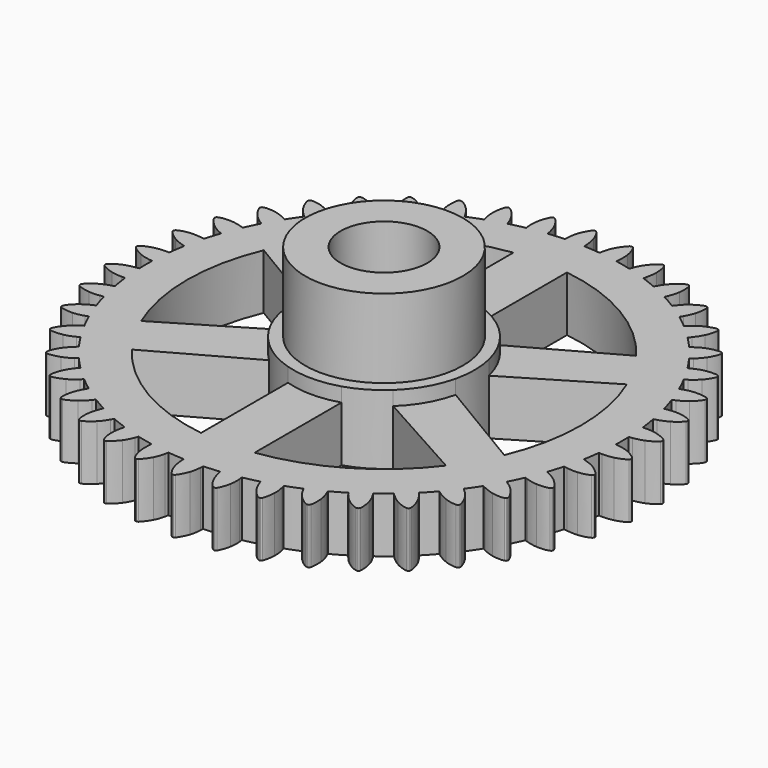
from build123d import *

# Parameters (mm, degrees)
F1_DEPTH  = 7
F2_R      = 4.1761413922
F3_DEPTH  = 25
F4_COUNT  = 42
F5_R      = 6.4823184413
F6_DEPTH  = 25
F7_R      = 30.25
F8_DEPTH  = 7
F10_DEPTH = 25
F11_R     = 5
F12_DEPTH = 1.8
F13_R     = 9.9
F13_R_2   = 5.0182312696
F14_DEPTH = 10
F15_R     = 10.7
F15_R_2   = 9.9
F16_DEPTH = 10
F17_R     = 12.382170164
F17_R_2   = 10
F18_DEPTH = 10
F17_R_3   = 5.5
F17_R_4   = 5.0182312696
F19_DEPTH = 91.7


with BuildPart() as f1:
    # F0 (on Top) → F1 (new body)
    with BuildSketch(Plane.XY):
        Polygon((0, 33.4545062297), (0, 33.4794496384), (-0.0728446466, 33.4794496384), align=None)
        with BuildLine():
            Line((0.0671612015, 33.4794496384), (0, 33.4794496384))
            Line((0, 33.4794496384), (0, 33.4545062297))
            Line((0, 33.4545062297), (0.2374699397, 33.3731919527))
            add(Edge.make_bspline(
                [(0.0671612015, 33.4794496384), (0.1192540142, 33.460955868), (0.1739978151, 33.4328680358), (0.2374699397, 33.3731919527)],
                knots=[0.0493061826, 0.0493061826, 0.0493061826, 0.0493061826, 0.1623395891, 0.1623395891, 0.1623395891, 0.1623395891], degree=3))
        make_face()
        Polygon((0.2374699397, 33.3731919527), (0, 33.4545062297), (0, 33.3731919527), align=None)
        with BuildLine():
            Line((0, 33.4545062297), (-0.0728446466, 33.4794496384))
            add(Edge.make_bspline(
                [(-0.0728446466, 33.4794496384), (-0.1154598232, 33.4657120562), (-0.1668077634, 33.4453793507), (-0.2365300603, 33.3731919527)],
                knots=[0.0695031824, 0.0695031824, 0.0695031824, 0.0695031824, 0.1811062055, 0.1811062055, 0.1811062055, 0.1811062055], degree=3))
            Line((-0.2365300603, 33.3731919527), (0, 33.3731919527))
            Line((0, 33.3731919527), (0, 33.4545062297))
        make_face()
        Polygon((0, 33.3731919527), (-0.2365300603, 33.3731919527), (0, 33.1028739042), align=None)
        with BuildLine():
            Line((0, 33.1028739042), (0.9666862315, 31.9980978966))
            add(Edge.make_bspline(
                [(0.2374699397, 33.3731919527), (0.4566645874, 33.1671065558), (0.7799529877, 32.5843005356), (0.9666862315, 31.9980978966)],
                knots=[0.1623395891, 0.1623395891, 0.1623395891, 0.1623395891, 0.5526891769, 0.5526891769, 0.5526891769, 0.5526891769], degree=3))
            Line((0.2374699397, 33.3731919527), (0, 33.3731919527))
            Line((0, 33.3731919527), (0, 33.1028739042))
        make_face()
        with BuildLine():
            add(Edge.make_bspline(
                [(-0.2365300603, 33.3731919527), (-0.4334827386, 33.1692758165), (-0.7770551927, 32.5515806531), (-0.9673137685, 31.9980978966)],
                knots=[0.1811062055, 0.1811062055, 0.1811062055, 0.1811062055, 0.4963642407, 0.4963642407, 0.4963642407, 0.4963642407], degree=3))
            Line((-0.9673137685, 31.9980978966), (0, 31.9980978966))
            Line((0, 31.9980978966), (0, 33.1028739042))
            Line((0, 33.1028739042), (-0.2365300603, 33.3731919527))
        make_face()
        Polygon((0, 31.9980978966), (0.9666862315, 31.9980978966), (0, 33.1028739042), align=None)
        with BuildLine():
            Line((0, 31.4007098089), (1.2083290596, 30.6544768805))
            add(Edge.make_bspline(
                [(0.9666862315, 31.9980978966), (1.1088668183, 31.5517572588), (1.1718801794, 31.1034474468), (1.2083290596, 30.6544768805)],
                knots=[0.5526891769, 0.5526891769, 0.5526891769, 0.5526891769, 0.8499053141, 0.8499053141, 0.8499053141, 0.8499053141], degree=3))
            Line((0.9666862315, 31.9980978966), (0, 31.9980978966))
            Line((0, 31.9980978966), (0, 31.4007098089))
        make_face()
        Polygon((0, 31.9980978966), (-0.9673137685, 31.9980978966), (0, 31.4007098089), align=None)
        with BuildLine():
            add(Edge.make_bspline(
                [(-0.9673137685, 31.9980978966), (-1.1457987858, 31.4788656937), (-1.1893575316, 31.0161446216), (-1.2146658644, 30.6501507258)],
                knots=[0.4963642407, 0.4963642407, 0.4963642407, 0.4963642407, 0.792113516, 0.792113516, 0.792113516, 0.792113516], degree=3))
            Line((-1.2146658644, 30.6501507258), (0, 30.6501507258))
            Line((0, 30.6501507258), (0, 31.4007098089))
            Line((0, 31.4007098089), (-0.9673137685, 31.9980978966))
        make_face()
        with BuildLine():
            Line((0, 30.6501507258), (1.2086794487, 30.6501507258))
            add(Edge.make_bspline(
                [(1.2083290596, 30.6544768805), (1.2084461294, 30.6530348357), (1.2085629252, 30.6515927842), (1.2086794487, 30.6501507258)],
                knots=[0.8499053141, 0.8499053141, 0.8499053141, 0.8499053141, 0.8508599401, 0.8508599401, 0.8508599401, 0.8508599401], degree=3))
            Line((1.2083290596, 30.6544768805), (0, 31.4007098089))
            Line((0, 31.4007098089), (0, 30.6501507258))
        make_face()
        with BuildLine():
            ThreePointArc((0, 30), (0.6251357368, 29.993486048), (1.25, 29.9739470207))
            add(Edge.make_bspline(
                [(1.2086794487, 30.6501507258), (1.2268837738, 30.4248597009), (1.2384418869, 30.1994033608), (1.25, 29.9739470207)],
                knots=[0.8508599401, 0.8508599401, 0.8508599401, 0.8508599401, 1, 1, 1, 1], degree=3))
            Line((1.2086794487, 30.6501507258), (0, 30.6501507258))
            Line((0, 30.6501507258), (0, 30))
        make_face()
        with BuildLine():
            add(Edge.make_bspline(
                [(-1.2146658644, 30.6501507258), (-1.2324554611, 30.3928882723), (-1.2412277305, 30.1834176465), (-1.25, 29.9739470207)],
                knots=[0.792113516, 0.792113516, 0.792113516, 0.792113516, 1, 1, 1, 1], degree=3))
            ThreePointArc((-1.25, 29.9739470207), (-0.6251357368, 29.993486048), (0, 30))
            Line((0, 30), (0, 30.6501507258))
            Line((0, 30.6501507258), (-1.2146658644, 30.6501507258))
        make_face()
    extrude(amount=F1_DEPTH)


with BuildPart() as f3:
    # F2 (on Top) → F3 (new body)
    with BuildSketch(Plane.XY):
        Circle(F2_R)
    extrude(amount=F3_DEPTH)

    # F5 (on face) → F6 (cut)
    with BuildSketch(Plane.XY.offset(25)):
        Circle(F5_R)
    extrude(amount=-F6_DEPTH, mode=Mode.SUBTRACT)


with BuildPart() as f4_1:
    # F4: instance of F1
    add(f1.part.rotate(Axis((0, 0, 25), (0, 0, 1)), 1 * 360 / F4_COUNT))


with BuildPart() as f4_2:
    # F4: instance of F1
    add(f1.part.rotate(Axis((0, 0, 25), (0, 0, 1)), 2 * 360 / F4_COUNT))


with BuildPart() as f4_3:
    # F4: instance of F1
    add(f1.part.rotate(Axis((0, 0, 25), (0, 0, 1)), 3 * 360 / F4_COUNT))


with BuildPart() as f4_4:
    # F4: instance of F1
    add(f1.part.rotate(Axis((0, 0, 25), (0, 0, 1)), 4 * 360 / F4_COUNT))


with BuildPart() as f4_5:
    # F4: instance of F1
    add(f1.part.rotate(Axis((0, 0, 25), (0, 0, 1)), 5 * 360 / F4_COUNT))


with BuildPart() as f4_6:
    # F4: instance of F1
    add(f1.part.rotate(Axis((0, 0, 25), (0, 0, 1)), 6 * 360 / F4_COUNT))


with BuildPart() as f4_7:
    # F4: instance of F1
    add(f1.part.rotate(Axis((0, 0, 25), (0, 0, 1)), 7 * 360 / F4_COUNT))


with BuildPart() as f4_8:
    # F4: instance of F1
    add(f1.part.rotate(Axis((0, 0, 25), (0, 0, 1)), 8 * 360 / F4_COUNT))


with BuildPart() as f4_9:
    # F4: instance of F1
    add(f1.part.rotate(Axis((0, 0, 25), (0, 0, 1)), 9 * 360 / F4_COUNT))


with BuildPart() as f4_10:
    # F4: instance of F1
    add(f1.part.rotate(Axis((0, 0, 25), (0, 0, 1)), 10 * 360 / F4_COUNT))


with BuildPart() as f4_11:
    # F4: instance of F1
    add(f1.part.rotate(Axis((0, 0, 25), (0, 0, 1)), 11 * 360 / F4_COUNT))


with BuildPart() as f4_12:
    # F4: instance of F1
    add(f1.part.rotate(Axis((0, 0, 25), (0, 0, 1)), 12 * 360 / F4_COUNT))


with BuildPart() as f4_13:
    # F4: instance of F1
    add(f1.part.rotate(Axis((0, 0, 25), (0, 0, 1)), 13 * 360 / F4_COUNT))


with BuildPart() as f4_14:
    # F4: instance of F1
    add(f1.part.rotate(Axis((0, 0, 25), (0, 0, 1)), 14 * 360 / F4_COUNT))


with BuildPart() as f4_15:
    # F4: instance of F1
    add(f1.part.rotate(Axis((0, 0, 25), (0, 0, 1)), 15 * 360 / F4_COUNT))


with BuildPart() as f4_16:
    # F4: instance of F1
    add(f1.part.rotate(Axis((0, 0, 25), (0, 0, 1)), 16 * 360 / F4_COUNT))


with BuildPart() as f4_17:
    # F4: instance of F1
    add(f1.part.rotate(Axis((0, 0, 25), (0, 0, 1)), 17 * 360 / F4_COUNT))


with BuildPart() as f4_18:
    # F4: instance of F1
    add(f1.part.rotate(Axis((0, 0, 25), (0, 0, 1)), 18 * 360 / F4_COUNT))


with BuildPart() as f4_19:
    # F4: instance of F1
    add(f1.part.rotate(Axis((0, 0, 25), (0, 0, 1)), 19 * 360 / F4_COUNT))


with BuildPart() as f4_20:
    # F4: instance of F1
    add(f1.part.rotate(Axis((0, 0, 25), (0, 0, 1)), 20 * 360 / F4_COUNT))


with BuildPart() as f4_21:
    # F4: instance of F1
    add(f1.part.rotate(Axis((0, 0, 25), (0, 0, 1)), 21 * 360 / F4_COUNT))


with BuildPart() as f4_22:
    # F4: instance of F1
    add(f1.part.rotate(Axis((0, 0, 25), (0, 0, 1)), 22 * 360 / F4_COUNT))


with BuildPart() as f4_23:
    # F4: instance of F1
    add(f1.part.rotate(Axis((0, 0, 25), (0, 0, 1)), 23 * 360 / F4_COUNT))


with BuildPart() as f4_24:
    # F4: instance of F1
    add(f1.part.rotate(Axis((0, 0, 25), (0, 0, 1)), 24 * 360 / F4_COUNT))


with BuildPart() as f4_25:
    # F4: instance of F1
    add(f1.part.rotate(Axis((0, 0, 25), (0, 0, 1)), 25 * 360 / F4_COUNT))


with BuildPart() as f4_26:
    # F4: instance of F1
    add(f1.part.rotate(Axis((0, 0, 25), (0, 0, 1)), 26 * 360 / F4_COUNT))


with BuildPart() as f4_27:
    # F4: instance of F1
    add(f1.part.rotate(Axis((0, 0, 25), (0, 0, 1)), 27 * 360 / F4_COUNT))


with BuildPart() as f4_28:
    # F4: instance of F1
    add(f1.part.rotate(Axis((0, 0, 25), (0, 0, 1)), 28 * 360 / F4_COUNT))


with BuildPart() as f4_29:
    # F4: instance of F1
    add(f1.part.rotate(Axis((0, 0, 25), (0, 0, 1)), 29 * 360 / F4_COUNT))


with BuildPart() as f4_30:
    # F4: instance of F1
    add(f1.part.rotate(Axis((0, 0, 25), (0, 0, 1)), 30 * 360 / F4_COUNT))


with BuildPart() as f4_31:
    # F4: instance of F1
    add(f1.part.rotate(Axis((0, 0, 25), (0, 0, 1)), 31 * 360 / F4_COUNT))


with BuildPart() as f4_32:
    # F4: instance of F1
    add(f1.part.rotate(Axis((0, 0, 25), (0, 0, 1)), 32 * 360 / F4_COUNT))


with BuildPart() as f4_33:
    # F4: instance of F1
    add(f1.part.rotate(Axis((0, 0, 25), (0, 0, 1)), 33 * 360 / F4_COUNT))


with BuildPart() as f4_34:
    # F4: instance of F1
    add(f1.part.rotate(Axis((0, 0, 25), (0, 0, 1)), 34 * 360 / F4_COUNT))


with BuildPart() as f4_35:
    # F4: instance of F1
    add(f1.part.rotate(Axis((0, 0, 25), (0, 0, 1)), 35 * 360 / F4_COUNT))


with BuildPart() as f4_36:
    # F4: instance of F1
    add(f1.part.rotate(Axis((0, 0, 25), (0, 0, 1)), 36 * 360 / F4_COUNT))


with BuildPart() as f4_37:
    # F4: instance of F1
    add(f1.part.rotate(Axis((0, 0, 25), (0, 0, 1)), 37 * 360 / F4_COUNT))


with BuildPart() as f4_38:
    # F4: instance of F1
    add(f1.part.rotate(Axis((0, 0, 25), (0, 0, 1)), 38 * 360 / F4_COUNT))


with BuildPart() as f4_39:
    # F4: instance of F1
    add(f1.part.rotate(Axis((0, 0, 25), (0, 0, 1)), 39 * 360 / F4_COUNT))


with BuildPart() as f4_40:
    # F4: instance of F1
    add(f1.part.rotate(Axis((0, 0, 25), (0, 0, 1)), 40 * 360 / F4_COUNT))


with BuildPart() as f4_41:
    # F4: instance of F1
    add(f1.part.rotate(Axis((0, 0, 25), (0, 0, 1)), 41 * 360 / F4_COUNT))


with BuildPart() as f1_1:
    add(f1.part)

    add(f4_1.part)  # F8 merges F4_1

    add(f4_2.part)  # F8 merges F4_2

    add(f4_3.part)  # F8 merges F4_3

    add(f4_4.part)  # F8 merges F4_4

    add(f4_5.part)  # F8 merges F4_5

    add(f4_6.part)  # F8 merges F4_6

    add(f4_7.part)  # F8 merges F4_7

    add(f4_8.part)  # F8 merges F4_8

    add(f4_9.part)  # F8 merges F4_9

    add(f4_10.part)  # F8 merges F4_10

    add(f4_11.part)  # F8 merges F4_11

    add(f4_12.part)  # F8 merges F4_12

    add(f4_13.part)  # F8 merges F4_13

    add(f4_14.part)  # F8 merges F4_14

    add(f4_15.part)  # F8 merges F4_15

    add(f4_16.part)  # F8 merges F4_16

    add(f4_17.part)  # F8 merges F4_17

    add(f4_18.part)  # F8 merges F4_18

    add(f4_19.part)  # F8 merges F4_19

    add(f4_20.part)  # F8 merges F4_20

    add(f4_21.part)  # F8 merges F4_21

    add(f4_22.part)  # F8 merges F4_22

    add(f4_23.part)  # F8 merges F4_23

    add(f4_24.part)  # F8 merges F4_24

    add(f4_25.part)  # F8 merges F4_25

    add(f4_26.part)  # F8 merges F4_26

    add(f4_27.part)  # F8 merges F4_27

    add(f4_28.part)  # F8 merges F4_28

    add(f4_29.part)  # F8 merges F4_29

    add(f4_30.part)  # F8 merges F4_30

    add(f4_31.part)  # F8 merges F4_31

    add(f4_32.part)  # F8 merges F4_32

    add(f4_33.part)  # F8 merges F4_33

    add(f4_34.part)  # F8 merges F4_34

    add(f4_35.part)  # F8 merges F4_35

    add(f4_36.part)  # F8 merges F4_36

    add(f4_37.part)  # F8 merges F4_37

    add(f4_38.part)  # F8 merges F4_38

    add(f4_39.part)  # F8 merges F4_39

    add(f4_40.part)  # F8 merges F4_40

    add(f4_41.part)  # F8 merges F4_41
    # F7 (on Top) → F8 (join)
    with BuildSketch(Plane.XY):
        Circle(F7_R)
    extrude(amount=F8_DEPTH)

    # F9 (on face) → F10 (cut)
    with BuildSketch(Plane.XY.offset(7)):
        with BuildLine():
            ThreePointArc((3.4, 10.9859000542), (5.7866942093, 9.9380164081), (7.8760958819, 8.3795652428))
            Line((7.8760958819, 8.3795652428), (19.9333428077, 15.0884672685))
            ThreePointArc((19.9333428077, 15.0884672685), (12.6306456486, 21.5746793835), (3.4, 24.7677209287))
            Line((3.4, 24.7677209287), (3.4, 10.9859000542))
        make_face()
        with BuildLine():
            ThreePointArc((-7.8760958819, 8.3795652428), (-5.7866942093, 9.9380164081), (-3.4, 10.9859000542))
            Line((-3.4, 10.9859000542), (-3.4, 24.7677209287))
            ThreePointArc((-3.4, 24.7677209287), (-12.6306456486, 21.5746793835), (-19.9333428077, 15.0884672685))
            Line((-19.9333428077, 15.0884672685), (-7.8760958819, 8.3795652428))
        make_face()
        with BuildLine():
            ThreePointArc((-11.1949643139, -2.631116495), (-11.5, 0), (-11.1949643139, 2.631116495))
            Line((-11.1949643139, 2.631116495), (-23.0336673625, 9.7185476195))
            ThreePointArc((-23.0336673625, 9.7185476195), (-25, 0), (-23.0336673625, -9.7185476195))
            Line((-23.0336673625, -9.7185476195), (-11.1949643139, -2.631116495))
        make_face()
        with BuildLine():
            Line((-3.4, -24.7677209287), (-3.4, -10.9859000542))
            ThreePointArc((-3.4, -10.9859000542), (-5.7866942093, -9.9380164081), (-7.8760958819, -8.3795652428))
            Line((-7.8760958819, -8.3795652428), (-19.9333428077, -15.0884672685))
            ThreePointArc((-19.9333428077, -15.0884672685), (-12.6306456486, -21.5746793835), (-3.4, -24.7677209287))
        make_face()
        with BuildLine():
            Line((19.9333428077, -15.0884672685), (7.8760958819, -8.3795652428))
            ThreePointArc((7.8760958819, -8.3795652428), (5.7866942093, -9.9380164081), (3.4, -10.9859000542))
            Line((3.4, -10.9859000542), (3.4, -24.7677209287))
            ThreePointArc((3.4, -24.7677209287), (12.6306456486, -21.5746793835), (19.9333428077, -15.0884672685))
        make_face()
        Polygon((6.8, 0), (6.8, 3.9259818305), (3.4, 5.8889727457), (0, 7.851963661), (-3.4, 5.8889727457), (-6.8, 3.9259818305), (-6.8, 0), (-6.8, -3.9259818305), (-3.4, -5.8889727457), (0, -7.851963661), (3.4, -5.8889727457), (6.8, -3.9259818305), align=None)
        with BuildLine():
            Line((23.0336673625, 9.7185476195), (11.1949643139, 2.631116495))
            ThreePointArc((11.1949643139, 2.631116495), (11.4234865433, 1.324369735), (11.5, 0))
            ThreePointArc((11.5, 0), (11.4234865433, -1.324369735), (11.1949643139, -2.631116495))
            Line((11.1949643139, -2.631116495), (23.0336673625, -9.7185476195))
            ThreePointArc((23.0336673625, -9.7185476195), (24.503486324, -4.9577371823), (25, 0))
            ThreePointArc((25, 0), (24.503486324, 4.9577371823), (23.0336673625, 9.7185476195))
        make_face()
    extrude(amount=-F10_DEPTH, mode=Mode.SUBTRACT)

    # F11 (on face) → F12 (join)
    with BuildSketch(Plane.XY.offset(7)):
        with BuildLine():
            ThreePointArc((11.1949643139, -2.631116495), (11.4234865433, -1.324369735), (11.5, 0))
            ThreePointArc((11.5, 0), (11.4234865433, 1.324369735), (11.1949643139, 2.631116495))
            ThreePointArc((11.1949643139, 2.631116495), (9.9592921435, 5.75), (7.8760958819, 8.3795652428))
            ThreePointArc((7.8760958819, 8.3795652428), (5.7866942093, 9.9380164081), (3.4, 10.9859000542))
            ThreePointArc((3.4, 10.9859000542), (0, 11.5), (-3.4, 10.9859000542))
            ThreePointArc((-3.4, 10.9859000542), (-5.7866942093, 9.9380164081), (-7.8760958819, 8.3795652428))
            ThreePointArc((-7.8760958819, 8.3795652428), (-9.9592921435, 5.75), (-11.1949643139, 2.631116495))
            ThreePointArc((-11.1949643139, 2.631116495), (-11.5, 0), (-11.1949643139, -2.631116495))
            ThreePointArc((-11.1949643139, -2.631116495), (-9.9592921435, -5.75), (-7.8760958819, -8.3795652428))
            ThreePointArc((-7.8760958819, -8.3795652428), (-5.7866942093, -9.9380164081), (-3.4, -10.9859000542))
            ThreePointArc((-3.4, -10.9859000542), (0, -11.5), (3.4, -10.9859000542))
            ThreePointArc((3.4, -10.9859000542), (5.7866942093, -9.9380164081), (7.8760958819, -8.3795652428))
            ThreePointArc((7.8760958819, -8.3795652428), (9.9592921435, -5.75), (11.1949643139, -2.631116495))
        make_face()
        Polygon((6.8, 3.9259818305), (6.8, -3.9259818305), (0, -7.851963661), (-6.8, -3.9259818305), (-6.8, 3.9259818305), (0, 7.851963661), align=None, mode=Mode.SUBTRACT)
        Polygon((0, -7.851963661), (6.8, -3.9259818305), (6.8, 3.9259818305), (0, 7.851963661), (-6.8, 3.9259818305), (-6.8, -3.9259818305), align=None)
        Circle(F11_R, mode=Mode.SUBTRACT)
    extrude(amount=F12_DEPTH)

    # F13 (on face) → F14 (join)
    with BuildSketch(Plane.XY.offset(8.8)):
        Circle(F13_R)
        Circle(F13_R_2, mode=Mode.SUBTRACT)
    extrude(amount=F14_DEPTH)

    # F15 (on face) → F16 (join)
    with BuildSketch(Plane.XY.offset(8.8)):
        Circle(F15_R)
        Circle(F15_R_2, mode=Mode.SUBTRACT)
    extrude(amount=F16_DEPTH)

    # F17 (on face) → F18 (cut, through all)
    with BuildSketch(Plane.XY.offset(18.8)):
        Circle(F17_R)
        Circle(F17_R_2, mode=Mode.SUBTRACT)
    extrude(amount=-F18_DEPTH, mode=Mode.SUBTRACT)

    # F17 (on face) → F19 (cut)
    with BuildSketch(Plane.XY.offset(18.8)):
        Circle(F17_R_3)
        Circle(F17_R_4, mode=Mode.SUBTRACT)
        Circle(F17_R_4)
    extrude(amount=-F19_DEPTH, mode=Mode.SUBTRACT)


solid = f1_1.part
